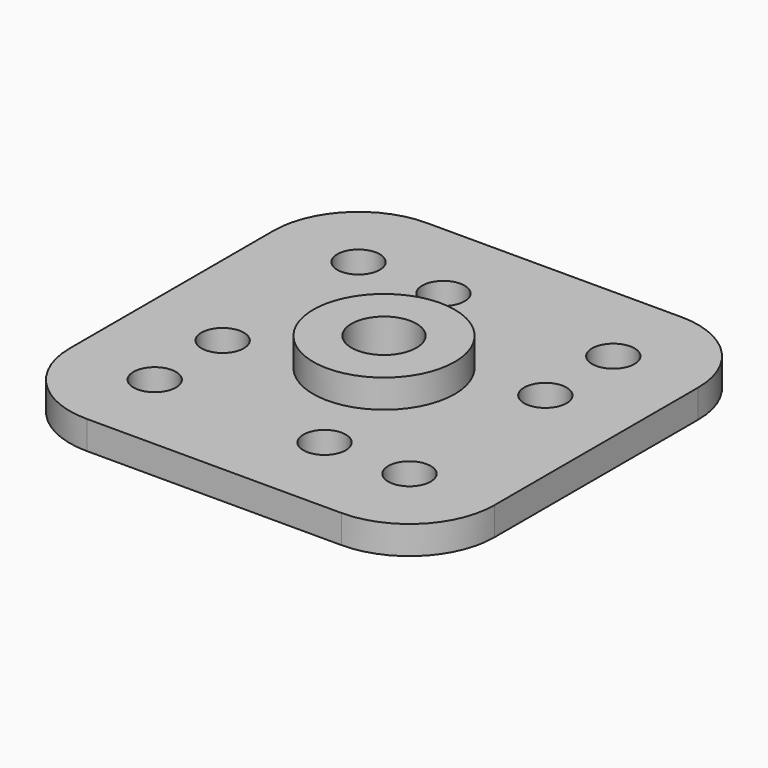
from build123d import *

# Parameters (mm, degrees)
F0_R            = 2.5
F0_R_2          = 1.15
F1_DEPTH        = 1
F2_W            = 15
F2_H            = 15
F2_R            = 5
F2_R_2          = 2.5
F2_R_3          = 1.15
F3_DEPTH        = 1
F4_R            = 3
F5_R            = 0.75
F6_DEPTH        = 25
F6_COPIES_COUNT = 4


# Not quite as in the source:
# - a pattern or mirror of a feature is missing from the dataset's text; its kind, count and spacing are read off the source's solid


with BuildPart() as f1:
    # F0 (on Top) → F1 (new body)
    with BuildSketch(Plane.XY):
        Circle(F0_R)
        Circle(F0_R_2, mode=Mode.SUBTRACT)
    extrude(amount=F1_DEPTH)

    # F2 (on face) → F3 (join)
    with BuildSketch(Plane(origin=(0, 0, 0), x_dir=(1, 0, 0), z_dir=(0, 0, -1))):
        Rectangle(F2_W, F2_H)
        Circle(F2_R, mode=Mode.SUBTRACT)
        Circle(F2_R)
        Circle(F2_R_2, mode=Mode.SUBTRACT)
        Circle(F2_R_2)
        Circle(F2_R_3, mode=Mode.SUBTRACT)
    extrude(amount=F3_DEPTH)

    # F4
    f4_edges = [f1.edges().sort_by_distance(p)[0] for p in [
        (-7.5, 7.5, -0.5),
        (7.5, 7.5, -0.5),
        (-7.5, -7.5, -0.5),
        (7.5, -7.5, -0.5),
    ]]
    fillet(f4_edges, radius=F4_R)

    # F5 (on face) → F6 (cut)
    with BuildSketch(Plane.XY):
        with Locations((-4.5, 4.5)):
            Circle(F5_R)
        with Locations((-1.5, 4.5)):
            Circle(F5_R)
    f6 = extrude(amount=-F6_DEPTH, mode=Mode.SUBTRACT)

    # F6_copies: F6 ×4 about axis
    f6_copies_axis = Axis((0, 0, 0), (0, 0, 1))
    for i in range(1, F6_COPIES_COUNT):
        add(f6.rotate(f6_copies_axis, i * 360 / F6_COPIES_COUNT), mode=Mode.SUBTRACT)


solid = f1.part
